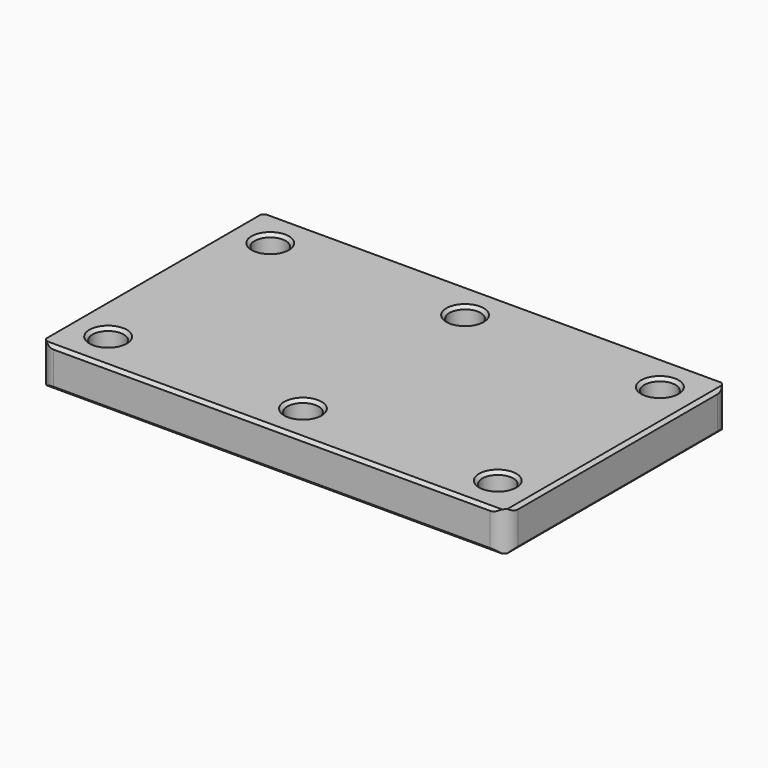
from build123d import *

# Parameters (mm, degrees)
F0_W        = 300
F0_H        = 180
F0_R        = 10
F1_DEPTH    = 25
F2_SIZE2    = 2
F2_SIZE     = 2
F3_SIZE2    = 2
F3_SIZE     = 2
F4_T1_DEPTH = 71


# Not quite as in the source:
# - a fillet or chamfer that OpenCascade refuses, or shapes differently, is made with other operations: its cross-section is extruded or revolved along the edge and cut away or added


with BuildPart() as f1:
    # F0 (on Top) → F1 (new body)
    with BuildSketch(Plane.XY):
        Rectangle(F0_W, F0_H)
        with Locations((-125, -65)):
            Circle(F0_R, mode=Mode.SUBTRACT)
        with Locations((0, -65)):
            Circle(F0_R, mode=Mode.SUBTRACT)
        with Locations((125, -65)):
            Circle(F0_R, mode=Mode.SUBTRACT)
        with Locations((-125, 65)):
            Circle(F0_R, mode=Mode.SUBTRACT)
        with Locations((0, 65)):
            Circle(F0_R, mode=Mode.SUBTRACT)
        with Locations((125, 65)):
            Circle(F0_R, mode=Mode.SUBTRACT)
    extrude(amount=F1_DEPTH)

    # F2
    f2_edges = [f1.edges().sort_by_distance(p)[0] for p in [
        (-135, -65, 25),
        (-135, 65, 25),
        (-10, -65, 25),
        (-10, 65, 25),
        (115, 65, 25),
        (115, -65, 25),
        (-150, 0, 25),
        (-150, 0, 0),
        (150, 0, 25),
        (150, 0, 0),
    ]]
    chamfer(f2_edges, length=F2_SIZE, length2=F2_SIZE2)

    # F3
    f3_edges = [f1.edges().sort_by_distance(p)[0] for p in [
        (0, -90, 25),
        (0, -90, 0),
        (0, 90, 25),
        (0, 90, 0),
    ]]
    chamfer(f3_edges, length=F3_SIZE, length2=F3_SIZE2)

    # F4: fillet of radius 10 on 4 edges, made by hand

    # F4_s2 → F4_t1 (cut)
    with BuildSketch(Plane.XY.offset(-23)):
        with BuildLine():
            ThreePointArc((150, -80), (147.0710678119, -87.0710678119), (140, -90))
            Line((140, -90), (150, -90))
            Line((150, -90), (150, -80))
        make_face()
        with BuildLine():
            ThreePointArc((-150, -80), (-147.0710678119, -87.0710678119), (-140, -90))
            Line((-140, -90), (-150, -90))
            Line((-150, -90), (-150, -80))
        make_face()
        with BuildLine():
            ThreePointArc((-140, 90), (-147.0710678119, 87.0710678119), (-150, 80))
            Line((-150, 80), (-150, 90))
            Line((-150, 90), (-140, 90))
        make_face()
        with BuildLine():
            ThreePointArc((140, 90), (147.0710678119, 87.0710678119), (150, 80))
            Line((150, 80), (150, 90))
            Line((150, 90), (140, 90))
        make_face()
    extrude(amount=F4_T1_DEPTH, mode=Mode.SUBTRACT)


solid = f1.part
